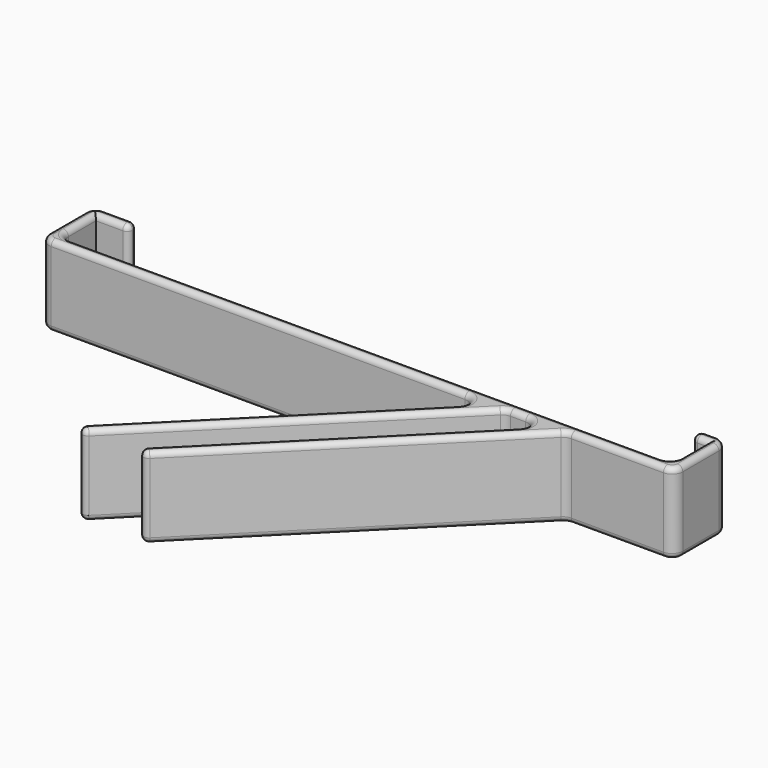
from build123d import *

# Parameters (mm, degrees)
F1_DEPTH      = 15
F2_R          = 0.99999
F3_R          = 2
F4_T1_DEPTH   = 62.6715828753
F4_T3_DEPTH   = 110
F4_T5_DEPTH   = 56.6715828753
F4_T7_DEPTH   = 6.4
F4_T9_DEPTH   = 7.50001
F4_T11_DEPTH  = 5.00002
F4_T13_DEPTH  = 4.50001
F4_T15_DEPTH  = 8.4
F4_T17_DEPTH  = 77.0294372515
F4_T19_DEPTH  = 56.6715828753
F4_T21_DEPTH  = 17.1715728753
F4_T23_DEPTH  = 5.0000200007
F4_T25_DEPTH  = 62.6715828753
F4_T27_DEPTH  = 5.0000199998
F4_T29_DEPTH  = 2.8284271247
F4_T32_ANGLE  = 90
F4_T34_ANGLE  = 90
F4_T36_ANGLE  = 90
F4_T38_ANGLE  = 90
F4_T40_ANGLE  = 90
F4_T42_ANGLE  = 90
F4_T44_ANGLE  = 90
F4_T46_ANGLE  = 90
F4_T48_ANGLE  = 90
F4_T50_ANGLE  = 135
F4_T52_ANGLE  = 90
F4_T54_ANGLE  = 90
F4_T56_ANGLE  = 45
F4_T58_ANGLE  = 90
F4_T60_ANGLE  = 90
F4_T62_ANGLE  = 45
F4_T64_ANGLE  = 90
F4_T66_ANGLE  = 135
F4_T68_ANGLE  = 90
F4_T70_ANGLE  = 90
F4_T72_ANGLE  = 90
F4_T74_ANGLE  = 90
F4_T76_ANGLE  = 90
F4_T78_ANGLE  = 90
F4_T80_ANGLE  = 90
F4_T82_ANGLE  = 90
F4_T84_ANGLE  = 90
F4_T86_ANGLE  = 135
F4_T88_ANGLE  = 90
F4_T90_ANGLE  = 90
F4_T92_ANGLE  = 45
F4_T94_ANGLE  = 90
F4_T96_ANGLE  = 90
F4_T98_ANGLE  = 45
F4_T100_ANGLE = 90
F4_T102_ANGLE = 135
F4_T107_DEPTH = 8.9
F4_T111_DEPTH = 10.00001
F4_T118_DEPTH = 8.9
F4_T122_DEPTH = 7.00001
F4_T129_DEPTH = 8.9
F4_T133_DEPTH = 10.00001
F4_T140_DEPTH = 8.9
F4_T144_DEPTH = 7.00001


# Not quite as in the source:
# - a fillet or chamfer that OpenCascade refuses, or shapes differently, is made with other operations: its cross-section is extruded or revolved along the edge and cut away or added
# - a fillet or chamfer is up to 0.001 mm smaller than in the source, because OpenCascade refuses the exact size
# - a feature names something its author has since deleted; it is built from what else it names


with BuildPart() as f1:
    # F0 (on Top) → F1 (new body)
    with BuildSketch(Plane.XY):
        Polygon((61.9649468476, 0.3016514366), (-52.0350531524, 0.3016514366), (-52.0350531524, -1.6983485634), (29.8228112239, -1.6983485634), (32.6512383486, -1.6983485634), (41.1365197229, -1.6983485634), (43.9649468476, -1.6983485634), (61.9649468476, -1.6983485634), align=None)
        Polygon((-52.0350531524, -1.6983485634), (-52.0350531524, 0.3016514366), (-52.0350531524, 8.7016514366), (-54.0350531524, 8.7016514366), (-54.0350531524, -1.6983485634), align=None)
        Polygon((61.9649468476, 8.7016514366), (61.9649468476, 0.3016514366), (61.9649468476, -1.6983485634), (63.9649468476, -1.6983485634), (63.9649468476, 8.7016514366), align=None)
        Polygon((-54.0350531524, 8.7016514366), (-52.0350531524, 8.7016514366), (-46.0350531524, 8.7016514366), (-46.0350531524, 10.7016514366), (-54.0350531524, 10.7016514366), align=None)
        Polygon((58.9649468476, 8.7016514366), (61.9649468476, 8.7016514366), (63.9649468476, 8.7016514366), (63.9649468476, 10.7016514366), (58.9649468476, 10.7016514366), align=None)
        Polygon((32.6512383486, -1.6983485634), (29.8228112239, -1.6983485634), (-12.6035956473, -44.1247554346), (-11.1893820849, -45.538968997), align=None)
        Polygon((0.124326414, -45.538968997), (43.9649468476, -1.6983485634), (41.1365197229, -1.6983485634), (-1.2898871483, -44.1247554346), align=None)
    extrude(amount=F1_DEPTH)

    # F2 (radius 1 in the source; OpenCascade refuses exactly that, so slightly less here)
    f2_edges = [f1.edges().sort_by_distance(p)[0] for p in [
        (58.964947, 10.701651, 7.5),
        (58.964947, 8.701651, 7.5),
        (-46.035053, 8.701651, 7.5),
        (-46.035053, 10.701651, 7.5),
        (0.124326, -45.538969, 7.5),
        (-1.289887, -44.124755, 7.5),
        (-11.189382, -45.538969, 7.5),
        (-12.603596, -44.124755, 7.5),
    ]]
    fillet(f2_edges, radius=F2_R)

    # F3
    f3_edges = [f1.edges().sort_by_distance(p)[0] for p in [
        (-54.035053, 10.701651, 7.5),
        (-54.035053, -1.698349, 7.5),
        (63.964947, -1.698349, 7.5),
        (63.964947, 10.701651, 7.5),
        (43.964947, -1.698349, 7.5),
        (41.13652, -1.698349, 7.5),
        (32.651238, -1.698349, 7.5),
        (29.822811, -1.698349, 7.5),
        (-52.035053, 0.301651, 7.5),
        (61.964947, 0.301651, 7.5),
    ]]
    fillet(f3_edges, radius=F3_R)

    # F4: fillet of radius 1 on 76 edges, made by hand

    # F4_s2 → F4_t1 (cut)
    with BuildSketch(Plane(origin=(-23.7679885343, -23.7679885343, 0), x_dir=(0, 0, 1), z_dir=(0.7071067812, 0.7071067812, 0))):
        with BuildLine():
            ThreePointArc((14, 32.2888258365), (14.7071067812, 31.9959326176), (15, 31.2888258365))
            Line((15, 31.2888258365), (15, 32.2888258365))
            Line((15, 32.2888258365), (14, 32.2888258365))
        make_face()
        with BuildLine():
            ThreePointArc((0, 31.2888258365), (0.2928932188, 31.9959326176), (1, 32.2888258365))
            Line((1, 32.2888258365), (0, 32.2888258365))
            Line((0, 32.2888258365), (0, 31.2888258365))
        make_face()
    extrude(amount=F4_T1_DEPTH, mode=Mode.SUBTRACT)

    # F4_s4 → F4_t3 (cut)
    with BuildSketch(Plane.YZ.offset(-50.0350531524)):
        with BuildLine():
            ThreePointArc((0.3016514366, 14), (0.0087582178, 14.7071067812), (-0.6983485634, 15))
            Line((-0.6983485634, 15), (0.3016514366, 15))
            Line((0.3016514366, 15), (0.3016514366, 14))
        make_face()
        with BuildLine():
            ThreePointArc((-0.6983485634, 0), (0.0087582178, 0.2928932188), (0.3016514366, 1))
            Line((0.3016514366, 1), (0.3016514366, 0))
            Line((0.3016514366, 0), (-0.6983485634, 0))
        make_face()
    extrude(amount=F4_T3_DEPTH, mode=Mode.SUBTRACT)

    # F4_s6 → F4_t5 (cut)
    with BuildSketch(Plane(origin=(16.3048720174, 16.3048720174, 0), x_dir=(0, 0, 1), z_dir=(-0.7071067812, -0.7071067812, 0))):
        with BuildLine():
            ThreePointArc((0, -31.2888258365), (0.2928932188, -30.5817190553), (1, -30.2888258365))
            Line((1, -30.2888258365), (0, -30.2888258365))
            Line((0, -30.2888258365), (0, -31.2888258365))
        make_face()
        with BuildLine():
            ThreePointArc((14, -30.2888258365), (14.7071067812, -30.5817190553), (15, -31.2888258365))
            Line((15, -31.2888258365), (15, -30.2888258365))
            Line((15, -30.2888258365), (14, -30.2888258365))
        make_face()
    extrude(amount=F4_T5_DEPTH, mode=Mode.SUBTRACT)

    # F4_s8 → F4_t7 (cut)
    with BuildSketch(Plane.XZ.offset(-8.7016514366)):
        with BuildLine():
            ThreePointArc((-53.0350531524, 0), (-52.3279463712, 0.2928932188), (-52.0350531524, 1))
            Line((-52.0350531524, 1), (-52.0350531524, 0))
            Line((-52.0350531524, 0), (-53.0350531524, 0))
        make_face()
        with BuildLine():
            ThreePointArc((62.9649468476, 0), (62.2578400664, 0.2928932188), (61.9649468476, 1))
            Line((61.9649468476, 1), (61.9649468476, 0))
            Line((61.9649468476, 0), (62.9649468476, 0))
        make_face()
        with BuildLine():
            ThreePointArc((-52.0350531524, 14), (-52.3279463712, 14.7071067812), (-53.0350531524, 15))
            Line((-53.0350531524, 15), (-52.0350531524, 15))
            Line((-52.0350531524, 15), (-52.0350531524, 14))
        make_face()
        with BuildLine():
            ThreePointArc((61.9649468476, 14), (62.2578400664, 14.7071067812), (62.9649468476, 15))
            Line((62.9649468476, 15), (61.9649468476, 15))
            Line((61.9649468476, 15), (61.9649468476, 14))
        make_face()
    extrude(amount=F4_T7_DEPTH, mode=Mode.SUBTRACT)

    # F4_s10 → F4_t9 (cut)
    with BuildSketch(Plane.YZ.offset(-52.0350531524)):
        with BuildLine():
            ThreePointArc((9.7016514366, 0), (8.9945446554, 0.2928932188), (8.7016514366, 1))
            Line((8.7016514366, 1), (8.7016514366, 0))
            Line((8.7016514366, 0), (9.7016514366, 0))
        make_face()
        with BuildLine():
            ThreePointArc((9.7016514366, 0), (10.4087582178, 0.2928932188), (10.7016514366, 1))
            Line((10.7016514366, 1), (10.7016514366, 0))
            Line((10.7016514366, 0), (9.7016514366, 0))
        make_face()
        with BuildLine():
            ThreePointArc((8.7016514366, 14), (8.9945446554, 14.7071067812), (9.7016514366, 15))
            Line((9.7016514366, 15), (8.7016514366, 15))
            Line((8.7016514366, 15), (8.7016514366, 14))
        make_face()
        with BuildLine():
            ThreePointArc((10.7016514366, 14), (10.4087582178, 14.7071067812), (9.7016514366, 15))
            Line((9.7016514366, 15), (10.7016514366, 15))
            Line((10.7016514366, 15), (10.7016514366, 14))
        make_face()
    extrude(amount=F4_T9_DEPTH, mode=Mode.SUBTRACT)

    # F4_s12 → F4_t11 (cut)
    with BuildSketch(Plane.XZ.offset(-12.2016614366)):
        with BuildLine():
            ThreePointArc((-47.0350531524, 0), (-46.3279463712, 0.2928932188), (-46.0350531524, 1))
            Line((-46.0350531524, 1), (-46.0350531524, 0))
            Line((-46.0350531524, 0), (-47.0350531524, 0))
        make_face()
        with BuildLine():
            ThreePointArc((59.9649468476, 0), (59.2578400664, 0.2928932188), (58.9649468476, 1))
            Line((58.9649468476, 1), (58.9649468476, 0))
            Line((58.9649468476, 0), (59.9649468476, 0))
        make_face()
        with BuildLine():
            ThreePointArc((-46.0350531524, 14), (-46.3279463712, 14.7071067812), (-47.0350531524, 15))
            Line((-47.0350531524, 15), (-46.0350531524, 15))
            Line((-46.0350531524, 15), (-46.0350531524, 14))
        make_face()
        with BuildLine():
            ThreePointArc((58.9649468476, 14), (59.2578400664, 14.7071067812), (59.9649468476, 15))
            Line((59.9649468476, 15), (58.9649468476, 15))
            Line((58.9649468476, 15), (58.9649468476, 14))
        make_face()
    extrude(amount=F4_T11_DEPTH, mode=Mode.SUBTRACT)

    # F4_s14 → F4_t13 (cut)
    with BuildSketch(Plane.YZ.offset(57.4649368476)):
        with BuildLine():
            ThreePointArc((9.7016514366, 0), (8.9945446554, 0.2928932188), (8.7016514366, 1))
            Line((8.7016514366, 1), (8.7016514366, 0))
            Line((8.7016514366, 0), (9.7016514366, 0))
        make_face()
        with BuildLine():
            ThreePointArc((9.7016514366, 0), (10.4087582178, 0.2928932188), (10.7016514366, 1))
            Line((10.7016514366, 1), (10.7016514366, 0))
            Line((10.7016514366, 0), (9.7016514366, 0))
        make_face()
        with BuildLine():
            ThreePointArc((8.7016514366, 14), (8.9945446554, 14.7071067812), (9.7016514366, 15))
            Line((9.7016514366, 15), (8.7016514366, 15))
            Line((8.7016514366, 15), (8.7016514366, 14))
        make_face()
        with BuildLine():
            ThreePointArc((10.7016514366, 14), (10.4087582178, 14.7071067812), (9.7016514366, 15))
            Line((9.7016514366, 15), (10.7016514366, 15))
            Line((10.7016514366, 15), (10.7016514366, 14))
        make_face()
    extrude(amount=F4_T13_DEPTH, mode=Mode.SUBTRACT)

    # F4_s16 → F4_t15 (cut)
    with BuildSketch(Plane.XZ.offset(-8.7016514366)):
        with BuildLine():
            ThreePointArc((-53.0350531524, 0), (-53.7421599336, 0.2928932188), (-54.0350531524, 1))
            Line((-54.0350531524, 1), (-54.0350531524, 0))
            Line((-54.0350531524, 0), (-53.0350531524, 0))
        make_face()
        with BuildLine():
            ThreePointArc((62.9649468476, 0), (63.6720536288, 0.2928932188), (63.9649468476, 1))
            Line((63.9649468476, 1), (63.9649468476, 0))
            Line((63.9649468476, 0), (62.9649468476, 0))
        make_face()
        with BuildLine():
            ThreePointArc((-54.0350531524, 14), (-53.7421599336, 14.7071067812), (-53.0350531524, 15))
            Line((-53.0350531524, 15), (-54.0350531524, 15))
            Line((-54.0350531524, 15), (-54.0350531524, 14))
        make_face()
        with BuildLine():
            ThreePointArc((63.9649468476, 14), (63.6720536288, 14.7071067812), (62.9649468476, 15))
            Line((62.9649468476, 15), (63.9649468476, 15))
            Line((63.9649468476, 15), (63.9649468476, 14))
        make_face()
    extrude(amount=F4_T15_DEPTH, mode=Mode.SUBTRACT)

    # F4_s18 → F4_t17 (cut)
    with BuildSketch(Plane.YZ.offset(-52.0350531524)):
        with BuildLine():
            ThreePointArc((-0.6983485634, 0), (-1.4054553446, 0.2928932188), (-1.6983485634, 1))
            Line((-1.6983485634, 1), (-1.6983485634, 0))
            Line((-1.6983485634, 0), (-0.6983485634, 0))
        make_face()
        with BuildLine():
            ThreePointArc((-1.6983485634, 14), (-1.4054553446, 14.7071067812), (-0.6983485634, 15))
            Line((-0.6983485634, 15), (-1.6983485634, 15))
            Line((-1.6983485634, 15), (-1.6983485634, 14))
        make_face()
    extrude(amount=F4_T17_DEPTH, mode=Mode.SUBTRACT)

    # F4_s20 → F4_t19 (cut)
    with BuildSketch(Plane(origin=(10.6480177679, 10.6480177679, 0), x_dir=(0, 0, 1), z_dir=(-0.7071067812, -0.7071067812, 0))):
        with BuildLine():
            ThreePointArc((0, -23.2888258365), (0.2928932188, -22.5817190553), (1, -22.2888258365))
            Line((1, -22.2888258365), (0, -22.2888258365))
            Line((0, -22.2888258365), (0, -23.2888258365))
        make_face()
        with BuildLine():
            ThreePointArc((14, -22.2888258365), (14.7071067812, -22.5817190553), (15, -23.2888258365))
            Line((15, -23.2888258365), (15, -22.2888258365))
            Line((15, -22.2888258365), (14, -22.2888258365))
        make_face()
    extrude(amount=F4_T19_DEPTH, mode=Mode.SUBTRACT)

    # F4_s22 → F4_t21 (cut)
    with BuildSketch(Plane.YZ.offset(44.7933739724)):
        with BuildLine():
            ThreePointArc((-0.6983485634, 0), (-1.4054553446, 0.2928932188), (-1.6983485634, 1))
            Line((-1.6983485634, 1), (-1.6983485634, 0))
            Line((-1.6983485634, 0), (-0.6983485634, 0))
        make_face()
        with BuildLine():
            ThreePointArc((-1.6983485634, 14), (-1.4054553446, 14.7071067812), (-0.6983485634, 15))
            Line((-0.6983485634, 15), (-1.6983485634, 15))
            Line((-1.6983485634, 15), (-1.6983485634, 14))
        make_face()
    extrude(amount=F4_T21_DEPTH, mode=Mode.SUBTRACT)

    # F4_s24 → F4_t23 (cut)
    with BuildSketch(Plane(origin=(14.6999126506, -14.6999126506, 0), x_dir=(0, 0, 1), z_dir=(0.7071067812, -0.7071067812, 0))):
        with BuildLine():
            ThreePointArc((0, 39.1130017356), (0.2928932188, 39.8201085167), (1, 40.1130017356))
            Line((1, 40.1130017356), (0, 40.1130017356))
            Line((0, 40.1130017356), (0, 39.1130017356))
        make_face()
        with BuildLine():
            ThreePointArc((14, 40.1130017356), (14.7071067812, 39.8201085167), (15, 39.1130017356))
            Line((15, 39.1130017356), (15, 40.1130017356))
            Line((15, 40.1130017356), (14, 40.1130017356))
        make_face()
    extrude(amount=F4_T23_DEPTH, mode=Mode.SUBTRACT)

    # F4_s26 → F4_t25 (cut)
    with BuildSketch(Plane(origin=(-29.4248427838, -29.4248427838, 0), x_dir=(0, 0, 1), z_dir=(0.7071067812, 0.7071067812, 0))):
        with BuildLine():
            ThreePointArc((0, 23.2888258365), (0.2928932188, 23.9959326176), (1, 24.2888258365))
            Line((1, 24.2888258365), (0, 24.2888258365))
            Line((0, 24.2888258365), (0, 23.2888258365))
        make_face()
        with BuildLine():
            ThreePointArc((14, 24.2888258365), (14.7071067812, 23.9959326176), (15, 23.2888258365))
            Line((15, 23.2888258365), (15, 24.2888258365))
            Line((15, 24.2888258365), (14, 24.2888258365))
        make_face()
    extrude(amount=F4_T25_DEPTH, mode=Mode.SUBTRACT)

    # F4_s28 → F4_t27 (cut)
    with BuildSketch(Plane(origin=(20.3567669004, -20.3567669004, 0), x_dir=(0, 0, 1), z_dir=(0.7071067812, -0.7071067812, 0))):
        with BuildLine():
            ThreePointArc((0, 31.1130017356), (0.2928932188, 31.8201085167), (1, 32.1130017356))
            Line((1, 32.1130017356), (0, 32.1130017356))
            Line((0, 32.1130017356), (0, 31.1130017356))
        make_face()
        with BuildLine():
            ThreePointArc((14, 32.1130017356), (14.7071067812, 31.8201085167), (15, 31.1130017356))
            Line((15, 31.1130017356), (15, 32.1130017356))
            Line((15, 32.1130017356), (14, 32.1130017356))
        make_face()
    extrude(amount=F4_T27_DEPTH, mode=Mode.SUBTRACT)

    # F4_s30 → F4_t29 (cut)
    with BuildSketch(Plane.YZ.offset(33.4796654734)):
        with BuildLine():
            ThreePointArc((-0.6983485634, 0), (-1.4054553446, 0.2928932188), (-1.6983485634, 1))
            Line((-1.6983485634, 1), (-1.6983485634, 0))
            Line((-1.6983485634, 0), (-0.6983485634, 0))
        make_face()
        with BuildLine():
            ThreePointArc((-1.6983485634, 14), (-1.4054553446, 14.7071067812), (-0.6983485634, 15))
            Line((-0.6983485634, 15), (-1.6983485634, 15))
            Line((-1.6983485634, 15), (-1.6983485634, 14))
        make_face()
    extrude(amount=F4_T29_DEPTH, mode=Mode.SUBTRACT)

    # F4_s31 → F4_t32 (revolve, cut)
    with BuildSketch(Plane.XZ.offset(-2.3016514366)):
        with BuildLine():
            ThreePointArc((-53.0350531524, 0), (-52.3279463712, 0.2928932188), (-52.0350531524, 1))
            Line((-52.0350531524, 1), (-52.0350531524, 0))
            Line((-52.0350531524, 0), (-53.0350531524, 0))
        make_face()
    revolve(axis=Axis((-50.0350531524, 2.3016514366, 0), (0, 0, 1)), revolution_arc=F4_T32_ANGLE, mode=Mode.SUBTRACT)

    # F4_s33 → F4_t34 (revolve, cut)
    with BuildSketch(Plane.YZ.offset(-47.0350431524)):
        with BuildLine():
            ThreePointArc((9.7016414366, 0), (8.9945411199, 0.2928967544), (8.7016514366, 1))
            Line((8.7016514366, 1), (8.7016514366, 0))
            Line((8.7016514366, 0), (9.7016414366, 0))
        make_face()
    revolve(axis=Axis((-47.0350431524, 9.7016414366, 0), (0, 0, 1)), revolution_arc=F4_T34_ANGLE, mode=Mode.SUBTRACT)

    # F4_s35 → F4_t36 (revolve, cut)
    with BuildSketch(Plane.YZ.offset(59.9649468476)):
        with BuildLine():
            ThreePointArc((-0.6983485634, 0), (0.0087582178, 0.2928932188), (0.3016514366, 1))
            Line((0.3016514366, 1), (0.3016514366, 0))
            Line((0.3016514366, 0), (-0.6983485634, 0))
        make_face()
    revolve(axis=Axis((59.9649468476, 2.3016514366, 0), (0, 0, 1)), revolution_arc=F4_T36_ANGLE, mode=Mode.SUBTRACT)

    # F4_s37 → F4_t38 (revolve, cut)
    with BuildSketch(Plane.XZ.offset(-9.7016614366)):
        with BuildLine():
            ThreePointArc((-47.0350431524, 0), (-46.3279428357, 0.2928967544), (-46.0350531524, 1))
            Line((-46.0350531524, 1), (-46.0350531524, 0))
            Line((-46.0350531524, 0), (-47.0350431524, 0))
        make_face()
    revolve(axis=Axis((-47.0350431524, 9.7016614366, 0), (0, 0, 1)), revolution_arc=F4_T38_ANGLE, mode=Mode.SUBTRACT)

    # F4_s39 → F4_t40 (revolve, cut)
    with BuildSketch(Plane.XZ.offset(-9.7016414366)):
        with BuildLine():
            ThreePointArc((59.9649368476, 0), (59.2578365309, 0.2928967544), (58.9649468476, 1))
            Line((58.9649468476, 1), (58.9649468476, 0))
            Line((58.9649468476, 0), (59.9649368476, 0))
        make_face()
    revolve(axis=Axis((59.9649368476, 9.7016414366, 0), (0, 0, 1)), revolution_arc=F4_T40_ANGLE, mode=Mode.SUBTRACT)

    # F4_s41 → F4_t42 (revolve, cut)
    with BuildSketch(Plane.YZ.offset(-52.0350531524)):
        with BuildLine():
            ThreePointArc((9.7016514366, 0), (10.4087582178, 0.2928932188), (10.7016514366, 1))
            Line((10.7016514366, 1), (10.7016514366, 0))
            Line((10.7016514366, 0), (9.7016514366, 0))
        make_face()
    revolve(axis=Axis((-52.0350531524, 8.7016514366, 0), (0, 0, 1)), revolution_arc=F4_T42_ANGLE, mode=Mode.SUBTRACT)

    # F4_s43 → F4_t44 (revolve, cut)
    with BuildSketch(Plane.YZ.offset(59.9649368476)):
        with BuildLine():
            ThreePointArc((9.7016614366, 0), (10.4087617533, 0.2928967544), (10.7016514366, 1))
            Line((10.7016514366, 1), (10.7016514366, 0))
            Line((10.7016514366, 0), (9.7016614366, 0))
        make_face()
    revolve(axis=Axis((59.9649368476, 9.7016614366, 0), (0, 0, 1)), revolution_arc=F4_T44_ANGLE, mode=Mode.SUBTRACT)

    # F4_s45 → F4_t46 (revolve, cut)
    with BuildSketch(Plane.XZ.offset(-0.3016514366)):
        with BuildLine():
            ThreePointArc((-53.0350531524, 0), (-53.7421599336, 0.2928932188), (-54.0350531524, 1))
            Line((-54.0350531524, 1), (-54.0350531524, 0))
            Line((-54.0350531524, 0), (-53.0350531524, 0))
        make_face()
    revolve(axis=Axis((-52.0350531524, 0.3016514366, 0), (0, 0, 1)), revolution_arc=F4_T46_ANGLE, mode=Mode.SUBTRACT)

    # F4_s47 → F4_t48 (revolve, cut)
    with BuildSketch(Plane.YZ.offset(61.9649468476)):
        with BuildLine():
            ThreePointArc((9.7016514366, 0), (10.4087582178, 0.2928932188), (10.7016514366, 1))
            Line((10.7016514366, 1), (10.7016514366, 0))
            Line((10.7016514366, 0), (9.7016514366, 0))
        make_face()
    revolve(axis=Axis((61.9649468476, 8.7016514366, 0), (0, 0, -1)), revolution_arc=F4_T48_ANGLE, mode=Mode.SUBTRACT)

    # F4_s49 → F4_t50 (revolve, cut)
    with BuildSketch(Plane.YZ.offset(24.9943840991)):
        with BuildLine():
            ThreePointArc((-0.6983485634, 0), (-1.4054553446, 0.2928932188), (-1.6983485634, 1))
            Line((-1.6983485634, 1), (-1.6983485634, 0))
            Line((-1.6983485634, 0), (-0.6983485634, 0))
        make_face()
    revolve(axis=Axis((24.9943840991, -3.6983485634, 0), (0, 0, -1)), revolution_arc=F4_T50_ANGLE, mode=Mode.SUBTRACT)

    # F4_s51 → F4_t52 (revolve, cut)
    with BuildSketch(Plane.XZ.offset(-0.3016514366)):
        with BuildLine():
            ThreePointArc((62.9649468476, 0), (63.6720536288, 0.2928932188), (63.9649468476, 1))
            Line((63.9649468476, 1), (63.9649468476, 0))
            Line((63.9649468476, 0), (62.9649468476, 0))
        make_face()
    revolve(axis=Axis((61.9649468476, 0.3016514366, 0), (0, 0, -1)), revolution_arc=F4_T52_ANGLE, mode=Mode.SUBTRACT)

    # F4_s53 → F4_t54 (revolve, cut)
    with BuildSketch(Plane(origin=(-27.6570758308, -27.6570758308, 0), x_dir=(0, 0, 1), z_dir=(0.7071067812, 0.7071067812, 0))):
        with BuildLine():
            ThreePointArc((0, 23.2888158365), (0.2928967544, 22.5817155197), (1, 22.2888258365))
            Line((1, 22.2888258365), (0, 22.2888258365))
            Line((0, 22.2888258365), (0, 23.2888158365))
        make_face()
    revolve(axis=Axis((-11.1893962271, -44.1247554346, 0), (0, 0, 1)), revolution_arc=F4_T54_ANGLE, mode=Mode.SUBTRACT)

    # F4_s55 → F4_t56 (revolve, cut)
    with BuildSketch(Plane.YZ.offset(44.7933739724)):
        with BuildLine():
            ThreePointArc((-0.6983485634, 0), (-1.4054553446, 0.2928932188), (-1.6983485634, 1))
            Line((-1.6983485634, 1), (-1.6983485634, 0))
            Line((-1.6983485634, 0), (-0.6983485634, 0))
        make_face()
    revolve(axis=Axis((44.7933739724, -3.6983485634, 0), (0, 0, 1)), revolution_arc=F4_T56_ANGLE, mode=Mode.SUBTRACT)

    # F4_s57 → F4_t58 (revolve, cut)
    with BuildSketch(Plane(origin=(16.4676937459, -16.4676937459, 0), x_dir=(0, 0, 1), z_dir=(-0.7071067812, 0.7071067812, 0))):
        with BuildLine():
            ThreePointArc((0, -39.1130117356), (0.2928967544, -39.8201120523), (1, -40.1130017356))
            Line((1, -40.1130017356), (0, -40.1130017356))
            Line((0, -40.1130017356), (0, -39.1130117356))
        make_face()
    revolve(axis=Axis((-11.1893820849, -44.1247695767, 0), (0, 0, 1)), revolution_arc=F4_T58_ANGLE, mode=Mode.SUBTRACT)

    # F4_s59 → F4_t60 (revolve, cut)
    with BuildSketch(Plane(origin=(22.1245479954, -22.1245479954, 0), x_dir=(0, 0, 1), z_dir=(-0.7071067812, 0.7071067812, 0))):
        with BuildLine():
            ThreePointArc((0, -31.1130117356), (0.2928967544, -31.8201120523), (1, -32.1130017356))
            Line((1, -32.1130017356), (0, -32.1130017356))
            Line((0, -32.1130017356), (0, -31.1130117356))
        make_face()
    revolve(axis=Axis((0.124326414, -44.1247695767, 0), (0, 0, 1)), revolution_arc=F4_T60_ANGLE, mode=Mode.SUBTRACT)

    # F4_s61 → F4_t62 (revolve, cut)
    with BuildSketch(Plane(origin=(14.890658455, 14.890658455, 0), x_dir=(0, 0, 1), z_dir=(-0.7071067812, -0.7071067812, 0))):
        with BuildLine():
            ThreePointArc((0, -23.2888258365), (0.2928932188, -23.9959326176), (1, -24.2888258365))
            Line((1, -24.2888258365), (0, -24.2888258365))
            Line((0, -24.2888258365), (0, -23.2888258365))
        make_face()
    revolve(axis=Axis((33.4796654734, -3.6983485634, 0), (0, 0, -1)), revolution_arc=F4_T62_ANGLE, mode=Mode.SUBTRACT)

    # F4_s63 → F4_t64 (revolve, cut)
    with BuildSketch(Plane(origin=(-22.0002215814, -22.0002215814, 0), x_dir=(0, 0, 1), z_dir=(0.7071067812, 0.7071067812, 0))):
        with BuildLine():
            ThreePointArc((0, 31.2888158365), (0.2928967544, 30.5817155197), (1, 30.2888258365))
            Line((1, 30.2888258365), (0, 30.2888258365))
            Line((0, 30.2888258365), (0, 31.2888158365))
        make_face()
    revolve(axis=Axis((0.1243122719, -44.1247554346, 0), (0, 0, 1)), revolution_arc=F4_T64_ANGLE, mode=Mode.SUBTRACT)

    # F4_s65 → F4_t66 (revolve, cut)
    with BuildSketch(Plane.YZ.offset(36.3080925981)):
        with BuildLine():
            ThreePointArc((-0.6983485634, 0), (-1.4054553446, 0.2928932188), (-1.6983485634, 1))
            Line((-1.6983485634, 1), (-1.6983485634, 0))
            Line((-1.6983485634, 0), (-0.6983485634, 0))
        make_face()
    revolve(axis=Axis((36.3080925981, -3.6983485634, 0), (0, 0, -1)), revolution_arc=F4_T66_ANGLE, mode=Mode.SUBTRACT)

    # F4_s67 → F4_t68 (revolve, cut)
    with BuildSketch(Plane.XZ.offset(-2.3016514366)):
        with BuildLine():
            ThreePointArc((-52.0350531524, 14), (-52.3279463712, 14.7071067812), (-53.0350531524, 15))
            Line((-53.0350531524, 15), (-52.0350531524, 15))
            Line((-52.0350531524, 15), (-52.0350531524, 14))
        make_face()
    revolve(axis=Axis((-50.0350531524, 2.3016514366, 15), (0, 0, 1)), revolution_arc=F4_T68_ANGLE, mode=Mode.SUBTRACT)

    # F4_s69 → F4_t70 (revolve, cut)
    with BuildSketch(Plane.YZ.offset(-47.0350431524)):
        with BuildLine():
            ThreePointArc((8.7016514366, 14), (8.9945411199, 14.7071032456), (9.7016414366, 14.9999999999))
            Line((9.7016414366, 14.9999999999), (8.7016514366, 15))
            Line((8.7016514366, 15), (8.7016514366, 14))
        make_face()
    revolve(axis=Axis((-47.0350431524, 9.7016414366, 15), (0, 0, 1)), revolution_arc=F4_T70_ANGLE, mode=Mode.SUBTRACT)

    # F4_s71 → F4_t72 (revolve, cut)
    with BuildSketch(Plane.YZ.offset(59.9649468476)):
        with BuildLine():
            ThreePointArc((0.3016514366, 14), (0.0087582178, 14.7071067812), (-0.6983485634, 15))
            Line((-0.6983485634, 15), (0.3016514366, 15))
            Line((0.3016514366, 15), (0.3016514366, 14))
        make_face()
    revolve(axis=Axis((59.9649468476, 2.3016514366, 15), (0, 0, 1)), revolution_arc=F4_T72_ANGLE, mode=Mode.SUBTRACT)

    # F4_s73 → F4_t74 (revolve, cut)
    with BuildSketch(Plane.XZ.offset(-9.7016614366)):
        with BuildLine():
            ThreePointArc((-46.0350531524, 14), (-46.3279428357, 14.7071032456), (-47.0350431524, 14.9999999999))
            Line((-47.0350431524, 14.9999999999), (-46.0350531524, 15))
            Line((-46.0350531524, 15), (-46.0350531524, 14))
        make_face()
    revolve(axis=Axis((-47.0350431524, 9.7016614366, 15), (0, 0, 1)), revolution_arc=F4_T74_ANGLE, mode=Mode.SUBTRACT)

    # F4_s75 → F4_t76 (revolve, cut)
    with BuildSketch(Plane.XZ.offset(-9.7016414366)):
        with BuildLine():
            ThreePointArc((58.9649468476, 14), (59.2578365309, 14.7071032456), (59.9649368476, 14.9999999999))
            Line((59.9649368476, 14.9999999999), (58.9649468476, 15))
            Line((58.9649468476, 15), (58.9649468476, 14))
        make_face()
    revolve(axis=Axis((59.9649368476, 9.7016414366, 15), (0, 0, 1)), revolution_arc=F4_T76_ANGLE, mode=Mode.SUBTRACT)

    # F4_s77 → F4_t78 (revolve, cut)
    with BuildSketch(Plane.YZ.offset(-52.0350531524)):
        with BuildLine():
            ThreePointArc((10.7016514366, 14), (10.4087582178, 14.7071067812), (9.7016514366, 15))
            Line((9.7016514366, 15), (10.7016514366, 15))
            Line((10.7016514366, 15), (10.7016514366, 14))
        make_face()
    revolve(axis=Axis((-52.0350531524, 8.7016514366, 15), (0, 0, 1)), revolution_arc=F4_T78_ANGLE, mode=Mode.SUBTRACT)

    # F4_s79 → F4_t80 (revolve, cut)
    with BuildSketch(Plane.YZ.offset(59.9649368476)):
        with BuildLine():
            ThreePointArc((10.7016514366, 14), (10.4087617533, 14.7071032456), (9.7016614366, 14.9999999999))
            Line((9.7016614366, 14.9999999999), (10.7016514366, 15))
            Line((10.7016514366, 15), (10.7016514366, 14))
        make_face()
    revolve(axis=Axis((59.9649368476, 9.7016614366, 15), (0, 0, 1)), revolution_arc=F4_T80_ANGLE, mode=Mode.SUBTRACT)

    # F4_s81 → F4_t82 (revolve, cut)
    with BuildSketch(Plane.XZ.offset(-0.3016514366)):
        with BuildLine():
            ThreePointArc((-54.0350531524, 14), (-53.7421599336, 14.7071067812), (-53.0350531524, 15))
            Line((-53.0350531524, 15), (-54.0350531524, 15))
            Line((-54.0350531524, 15), (-54.0350531524, 14))
        make_face()
    revolve(axis=Axis((-52.0350531524, 0.3016514366, 15), (0, 0, 1)), revolution_arc=F4_T82_ANGLE, mode=Mode.SUBTRACT)

    # F4_s83 → F4_t84 (revolve, cut)
    with BuildSketch(Plane.YZ.offset(61.9649468476)):
        with BuildLine():
            ThreePointArc((10.7016514366, 14), (10.4087582178, 14.7071067812), (9.7016514366, 15))
            Line((9.7016514366, 15), (10.7016514366, 15))
            Line((10.7016514366, 15), (10.7016514366, 14))
        make_face()
    revolve(axis=Axis((61.9649468476, 8.7016514366, 15), (0, 0, -1)), revolution_arc=F4_T84_ANGLE, mode=Mode.SUBTRACT)

    # F4_s85 → F4_t86 (revolve, cut)
    with BuildSketch(Plane.YZ.offset(24.9943840991)):
        with BuildLine():
            ThreePointArc((-1.6983485634, 14), (-1.4054553446, 14.7071067812), (-0.6983485634, 15))
            Line((-0.6983485634, 15), (-1.6983485634, 15))
            Line((-1.6983485634, 15), (-1.6983485634, 14))
        make_face()
    revolve(axis=Axis((24.9943840991, -3.6983485634, 15), (0, 0, -1)), revolution_arc=F4_T86_ANGLE, mode=Mode.SUBTRACT)

    # F4_s87 → F4_t88 (revolve, cut)
    with BuildSketch(Plane.XZ.offset(-0.3016514366)):
        with BuildLine():
            ThreePointArc((63.9649468476, 14), (63.6720536288, 14.7071067812), (62.9649468476, 15))
            Line((62.9649468476, 15), (63.9649468476, 15))
            Line((63.9649468476, 15), (63.9649468476, 14))
        make_face()
    revolve(axis=Axis((61.9649468476, 0.3016514366, 15), (0, 0, -1)), revolution_arc=F4_T88_ANGLE, mode=Mode.SUBTRACT)

    # F4_s89 → F4_t90 (revolve, cut)
    with BuildSketch(Plane(origin=(-27.6570758308, -27.6570758308, 0), x_dir=(0, 0, 1), z_dir=(0.7071067812, 0.7071067812, 0))):
        with BuildLine():
            ThreePointArc((14, 22.2888258365), (14.7071032456, 22.5817155197), (14.9999999999, 23.2888158365))
            Line((14.9999999999, 23.2888158365), (15, 22.2888258365))
            Line((15, 22.2888258365), (14, 22.2888258365))
        make_face()
    revolve(axis=Axis((-11.1893962271, -44.1247554346, 15), (0, 0, 1)), revolution_arc=F4_T90_ANGLE, mode=Mode.SUBTRACT)

    # F4_s91 → F4_t92 (revolve, cut)
    with BuildSketch(Plane.YZ.offset(44.7933739724)):
        with BuildLine():
            ThreePointArc((-1.6983485634, 14), (-1.4054553446, 14.7071067812), (-0.6983485634, 15))
            Line((-0.6983485634, 15), (-1.6983485634, 15))
            Line((-1.6983485634, 15), (-1.6983485634, 14))
        make_face()
    revolve(axis=Axis((44.7933739724, -3.6983485634, 15), (0, 0, 1)), revolution_arc=F4_T92_ANGLE, mode=Mode.SUBTRACT)

    # F4_s93 → F4_t94 (revolve, cut)
    with BuildSketch(Plane(origin=(16.4676937459, -16.4676937459, 0), x_dir=(0, 0, 1), z_dir=(-0.7071067812, 0.7071067812, 0))):
        with BuildLine():
            ThreePointArc((14, -40.1130017356), (14.7071032456, -39.8201120523), (15, -39.1130117356))
            Line((15, -39.1130117356), (15, -40.1130017356))
            Line((15, -40.1130017356), (14, -40.1130017356))
        make_face()
    revolve(axis=Axis((-11.1893820849, -44.1247695767, 15), (0, 0, 1)), revolution_arc=F4_T94_ANGLE, mode=Mode.SUBTRACT)

    # F4_s95 → F4_t96 (revolve, cut)
    with BuildSketch(Plane(origin=(22.1245479954, -22.1245479954, 0), x_dir=(0, 0, 1), z_dir=(-0.7071067812, 0.7071067812, 0))):
        with BuildLine():
            ThreePointArc((14, -32.1130017356), (14.7071032456, -31.8201120523), (15, -31.1130117356))
            Line((15, -31.1130117356), (15, -32.1130017356))
            Line((15, -32.1130017356), (14, -32.1130017356))
        make_face()
    revolve(axis=Axis((0.124326414, -44.1247695767, 15), (0, 0, 1)), revolution_arc=F4_T96_ANGLE, mode=Mode.SUBTRACT)

    # F4_s97 → F4_t98 (revolve, cut)
    with BuildSketch(Plane(origin=(14.890658455, 14.890658455, 0), x_dir=(0, 0, 1), z_dir=(-0.7071067812, -0.7071067812, 0))):
        with BuildLine():
            ThreePointArc((14, -24.2888258365), (14.7071067812, -23.9959326176), (15, -23.2888258365))
            Line((15, -23.2888258365), (15, -24.2888258365))
            Line((15, -24.2888258365), (14, -24.2888258365))
        make_face()
    revolve(axis=Axis((33.4796654734, -3.6983485634, 15), (0, 0, -1)), revolution_arc=F4_T98_ANGLE, mode=Mode.SUBTRACT)

    # F4_s99 → F4_t100 (revolve, cut)
    with BuildSketch(Plane(origin=(-22.0002215814, -22.0002215814, 0), x_dir=(0, 0, 1), z_dir=(0.7071067812, 0.7071067812, 0))):
        with BuildLine():
            ThreePointArc((14, 30.2888258365), (14.7071032456, 30.5817155197), (15, 31.2888158365))
            Line((15, 31.2888158365), (15, 30.2888258365))
            Line((15, 30.2888258365), (14, 30.2888258365))
        make_face()
    revolve(axis=Axis((0.1243122719, -44.1247554346, 15), (0, 0, 1)), revolution_arc=F4_T100_ANGLE, mode=Mode.SUBTRACT)

    # F4_s101 → F4_t102 (revolve, cut)
    with BuildSketch(Plane.YZ.offset(36.3080925981)):
        with BuildLine():
            ThreePointArc((-1.6983485634, 14), (-1.4054553446, 14.7071067812), (-0.6983485634, 15))
            Line((-0.6983485634, 15), (-1.6983485634, 15))
            Line((-1.6983485634, 15), (-1.6983485634, 14))
        make_face()
    revolve(axis=Axis((36.3080925981, -3.6983485634, 15), (0, 0, -1)), revolution_arc=F4_T102_ANGLE, mode=Mode.SUBTRACT)


with BuildPart() as f4_tool105:
    # F4_s106 → F4_t107 (new body)
    with BuildSketch(Plane.XZ.offset(-2.3016514366)):
        with BuildLine():
            ThreePointArc((-53.0350531524, 0), (-52.3279463712, 0.2928932188), (-52.0350531524, 1))
            Line((-52.0350531524, 1), (-52.0350531524, 0))
            Line((-52.0350531524, 0), (-53.0350531524, 0))
        make_face()
    extrude(amount=-F4_T107_DEPTH)

    split(bisect_by=Plane.XZ.offset(-8.7016514366), keep=Keep.BOTTOM)


with BuildPart() as f4_tool109:
    # F4_s110 → F4_t111 (new body)
    with BuildSketch(Plane.YZ.offset(-54.5350531524)):
        with BuildLine():
            ThreePointArc((9.7016514366, 0), (8.9945446554, 0.2928932188), (8.7016514366, 1))
            Line((8.7016514366, 1), (8.7016514366, 0))
            Line((8.7016514366, 0), (9.7016514366, 0))
        make_face()
    extrude(amount=F4_T111_DEPTH)

    split(bisect_by=Plane.YZ.offset(-52.0350531524), keep=Keep.BOTTOM)


with BuildPart() as f4_tool105_1:
    add(f4_tool105.part)

    # F4_t113: intersect F4_tool109
    add(f4_tool109.part, mode=Mode.INTERSECT)


with BuildPart() as f1_1:
    add(f1.part)

    # F4_t103: cut F4_tool105
    add(f4_tool105_1.part, mode=Mode.SUBTRACT)


with BuildPart() as f4_tool116:
    # F4_s117 → F4_t118 (new body)
    with BuildSketch(Plane.XZ.offset(-11.2016514366)):
        with BuildLine():
            ThreePointArc((62.9649468476, 0), (62.2578400664, 0.2928932188), (61.9649468476, 1))
            Line((61.9649468476, 1), (61.9649468476, 0))
            Line((61.9649468476, 0), (62.9649468476, 0))
        make_face()
    extrude(amount=F4_T118_DEPTH)

    split(bisect_by=Plane.XZ.offset(-8.7016514366), keep=Keep.BOTTOM)


with BuildPart() as f4_tool120:
    # F4_s121 → F4_t122 (new body)
    with BuildSketch(Plane.YZ.offset(57.4649368476)):
        with BuildLine():
            ThreePointArc((9.7016514366, 0), (8.9945446554, 0.2928932188), (8.7016514366, 1))
            Line((8.7016514366, 1), (8.7016514366, 0))
            Line((8.7016514366, 0), (9.7016514366, 0))
        make_face()
    extrude(amount=F4_T122_DEPTH)

    split(bisect_by=Plane.YZ.offset(61.9649468476), keep=Keep.TOP)


with BuildPart() as f4_tool116_1:
    add(f4_tool116.part)

    # F4_t124: intersect F4_tool120
    add(f4_tool120.part, mode=Mode.INTERSECT)


with BuildPart() as f1_2:
    add(f1_1.part)

    # F4_t114: cut F4_tool116
    add(f4_tool116_1.part, mode=Mode.SUBTRACT)


with BuildPart() as f4_tool127:
    # F4_s128 → F4_t129 (new body)
    with BuildSketch(Plane.XZ.offset(-2.3016514366)):
        with BuildLine():
            ThreePointArc((-52.0350531524, 14), (-52.3279463712, 14.7071067812), (-53.0350531524, 15))
            Line((-53.0350531524, 15), (-52.0350531524, 15))
            Line((-52.0350531524, 15), (-52.0350531524, 14))
        make_face()
    extrude(amount=-F4_T129_DEPTH)

    split(bisect_by=Plane.XZ.offset(-8.7016514366), keep=Keep.BOTTOM)


with BuildPart() as f4_tool131:
    # F4_s132 → F4_t133 (new body)
    with BuildSketch(Plane.YZ.offset(-54.5350531524)):
        with BuildLine():
            ThreePointArc((8.7016514366, 14), (8.9945446554, 14.7071067812), (9.7016514366, 15))
            Line((9.7016514366, 15), (8.7016514366, 15))
            Line((8.7016514366, 15), (8.7016514366, 14))
        make_face()
    extrude(amount=F4_T133_DEPTH)

    split(bisect_by=Plane.YZ.offset(-52.0350531524), keep=Keep.BOTTOM)


with BuildPart() as f4_tool127_1:
    add(f4_tool127.part)

    # F4_t135: intersect F4_tool131
    add(f4_tool131.part, mode=Mode.INTERSECT)


with BuildPart() as f1_3:
    add(f1_2.part)

    # F4_t125: cut F4_tool127
    add(f4_tool127_1.part, mode=Mode.SUBTRACT)


with BuildPart() as f4_tool138:
    # F4_s139 → F4_t140 (new body)
    with BuildSketch(Plane.XZ.offset(-11.2016514366)):
        with BuildLine():
            ThreePointArc((61.9649468476, 14), (62.2578400664, 14.7071067812), (62.9649468476, 15))
            Line((62.9649468476, 15), (61.9649468476, 15))
            Line((61.9649468476, 15), (61.9649468476, 14))
        make_face()
    extrude(amount=F4_T140_DEPTH)

    split(bisect_by=Plane.XZ.offset(-8.7016514366), keep=Keep.BOTTOM)


with BuildPart() as f4_tool142:
    # F4_s143 → F4_t144 (new body)
    with BuildSketch(Plane.YZ.offset(57.4649368476)):
        with BuildLine():
            ThreePointArc((8.7016514366, 14), (8.9945446554, 14.7071067812), (9.7016514366, 15))
            Line((9.7016514366, 15), (8.7016514366, 15))
            Line((8.7016514366, 15), (8.7016514366, 14))
        make_face()
    extrude(amount=F4_T144_DEPTH)

    split(bisect_by=Plane.YZ.offset(61.9649468476), keep=Keep.TOP)


with BuildPart() as f4_tool138_1:
    add(f4_tool138.part)

    # F4_t146: intersect F4_tool142
    add(f4_tool142.part, mode=Mode.INTERSECT)


with BuildPart() as f1_4:
    add(f1_3.part)

    # F4_t136: cut F4_tool138
    add(f4_tool138_1.part, mode=Mode.SUBTRACT)


solid = f1_4.part
